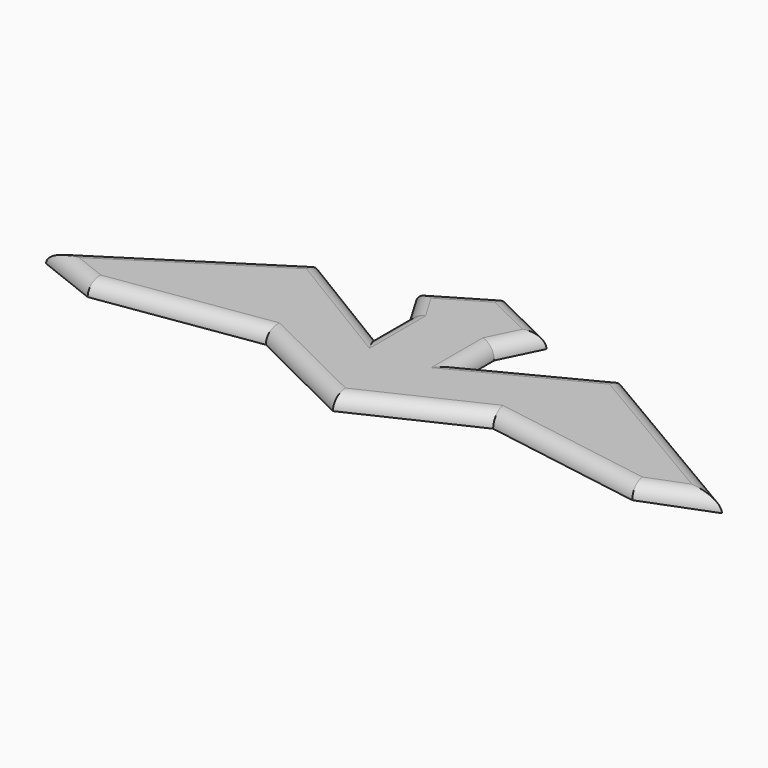
from build123d import *

# Parameters (mm, degrees)
F1_DEPTH = 2.54
F2_R     = 2.53999


# Not quite as in the source:
# - a fillet or chamfer is up to 0.001 mm smaller than in the source, because OpenCascade refuses the exact size


with BuildPart() as f1:
    # F0 (on Top) → F1 (new body)
    with BuildSketch(Plane.XY):
        Polygon((-27.0982775837, 20.9077224135), (-59.8030947149, 0), (-48.823621124, -4.3217078783), (-20.0901012868, 0), (0, -9.9282488227), (21.0245233029, 0), (49.9916523695, -4.7889198177), (62.3727589846, 0), (28.4999143332, 19.9733003974), (8.1038610589, 9.461035952), (8.1038610589, 16.395563461), (11.6802928969, 23.7109921873), (0, 29.4213576296), (-11.2130800262, 22.7765701711), (-7.4753868394, 16.4692122489), (-7.4753868394, 8.9938249439), align=None)
    extrude(amount=F1_DEPTH)

    # F2 (radius 2.54 in the source; OpenCascade refuses exactly that, so slightly less here)
    f2_edges = [f1.edges().sort_by_distance(p)[0] for p in [
        (-43.450686, 10.453861, 2.54),
        (-17.286832, 14.950774, 2.54),
        (-7.475387, 12.731519, 2.54),
        (-9.344233, 19.622891, 2.54),
        (-5.60654, 26.098964, 2.54),
        (5.840146, 26.566175, 2.54),
        (9.892077, 20.053278, 2.54),
        (8.103861, 12.9283, 2.54),
        (18.301888, 14.717168, 2.54),
        (45.436337, 9.98665, 2.54),
        (-54.313358, -2.160854, 2.54),
        (-34.456861, -2.160854, 2.54),
        (-10.045051, -4.964124, 2.54),
        (10.512262, -4.964124, 2.54),
        (35.508088, -2.39446, 2.54),
        (56.182206, -2.39446, 2.54),
    ]]
    fillet(f2_edges, radius=F2_R)


solid = f1.part
